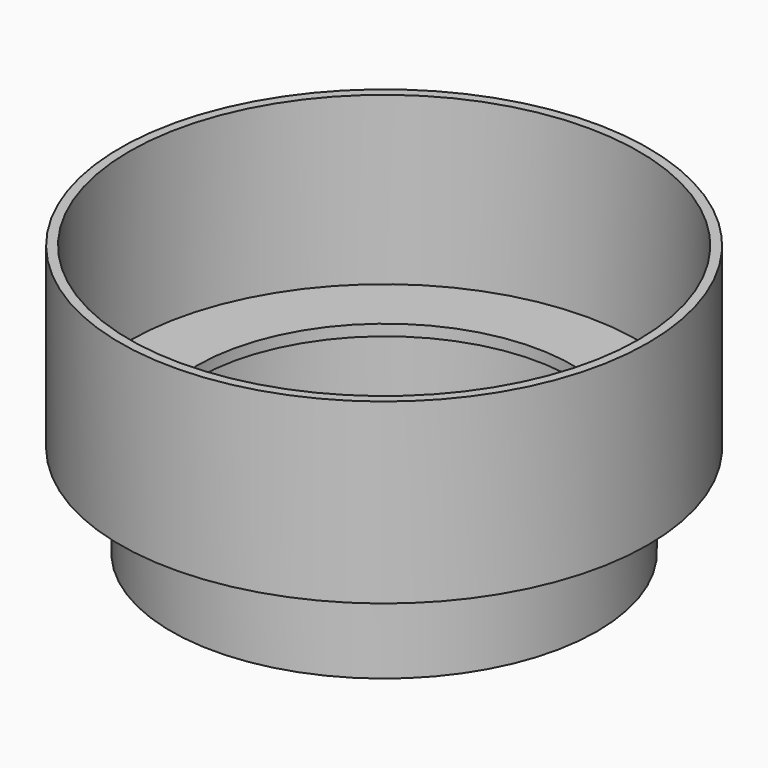
from build123d import *

# Parameters (mm, degrees)
F0_R     = 57.5
F0_R_2   = 55.5
F1_DEPTH = 25
F2_R     = 57.5
F2_R_2   = 55.5
F2_R_3   = 50.75
F3_DEPTH = 3
F2_R_4   = 71.25
F4_DEPTH = 3
F5_R     = 71.25
F5_R_2   = 68.75
F6_DEPTH = 45


with BuildPart() as f1:
    # F0 (on Top) → F1 (new body)
    with BuildSketch(Plane.XY):
        Circle(F0_R)
        Circle(F0_R_2, mode=Mode.SUBTRACT)
    extrude(amount=F1_DEPTH)

    # F2 (on face) → F3 (join)
    with BuildSketch(Plane.XY.offset(25)):
        Circle(F2_R)
        Circle(F2_R_2, mode=Mode.SUBTRACT)
        Circle(F2_R_2)
        with Locations((0.2079256644, 0.1388053244)):
            Circle(F2_R_3, mode=Mode.SUBTRACT)
    extrude(amount=F3_DEPTH)

    # F2 (on face) → F4 (join)
    with BuildSketch(Plane.XY.offset(25)):
        Circle(F2_R_4)
        Circle(F2_R, mode=Mode.SUBTRACT)
    extrude(amount=F4_DEPTH)

    # F5 (on face) → F6 (join)
    with BuildSketch(Plane.XY.offset(28)):
        Circle(F5_R)
        Circle(F5_R_2, mode=Mode.SUBTRACT)
    extrude(amount=F6_DEPTH)


solid = f1.part
